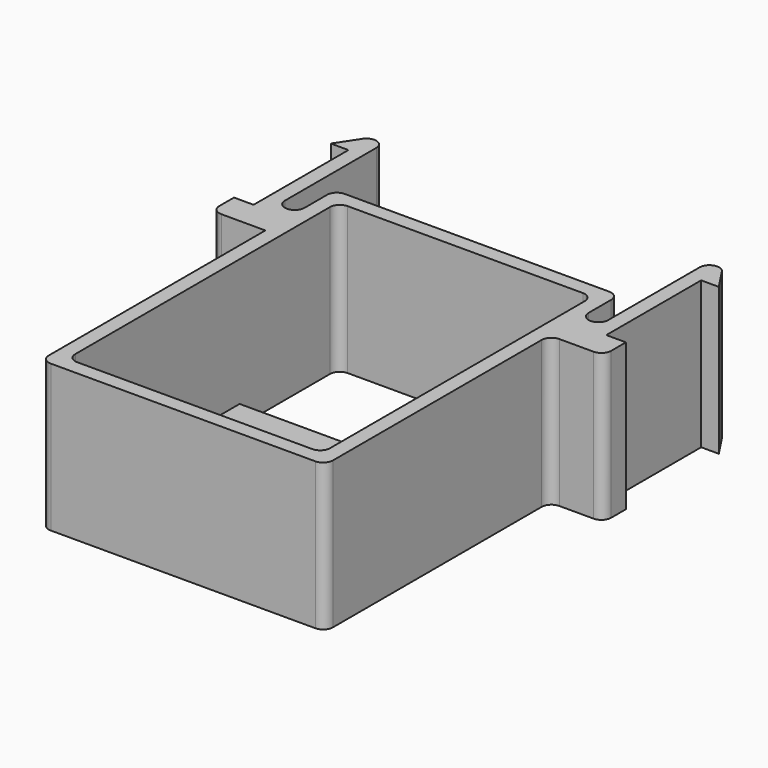
from build123d import *

# Parameters (mm, degrees)
F0_W     = 2
F0_H     = 4
F0_H_2   = 2.8740456328
F1_DEPTH = 15
F2_R     = 0.99999
F0_W_2   = 26
F0_H_3   = 7
F3_DEPTH = 2


# Not quite as in the source:
# - a fillet or chamfer is up to 0.001 mm smaller than in the source, because OpenCascade refuses the exact size


with BuildPart() as f1:
    # F0 (on Top) → F1 (new body)
    with BuildSketch(Plane.XY):
        Polygon((14.5, 18.75), (-14.5, 18.75), (-14.5, 13.8759543672), (-14.5, 9.8759543672), (-14.5, -18.75), (14.5, -18.75), (14.5, 9.8759543672), (14.5, 13.8759543672), align=None)
        Polygon((-13, 4.7144976147), (-13, 17.25), (13, 17.25), (13, 4.7144976147), (13, -2.2855023853), (13, -17.25), (-13, -17.25), (-13, -2.2855023853), align=None, mode=Mode.SUBTRACT)
        with Locations((-15.5, 11.8759543672)):
            Rectangle(F0_W, F0_H)
        Polygon((-16.5, 9.8759543672), (-16.5, 13.8759543672), (-16.5, 29.8609879265), (-19.8, 24.85), (-18, 24.85), (-18, 12.75), (-18, 9.8759543672), align=None)
        with Locations((15.5, 11.8759543672)):
            Rectangle(F0_W, F0_H)
        Polygon((16.5, 29.8609879265), (16.5, 13.8759543672), (16.5, 9.8759543672), (18, 9.8759543672), (18, 12.75), (18, 24.85), (19.8, 24.85), align=None)
        with Locations((-19, 11.3129771836)):
            Rectangle(F0_W, F0_H_2)
        with Locations((19, 11.3129771836)):
            Rectangle(F0_W, F0_H_2)
    extrude(amount=F1_DEPTH)

    # F2 (radius 1 in the source; OpenCascade refuses exactly that, so slightly less here)
    f2_edges = [f1.edges().sort_by_distance(p)[0] for p in [
        (-14.5, 18.75, 7.5),
        (-20, 9.875954, 7.5),
        (14.5, 18.75, 7.5),
        (20, 9.875954, 7.5),
        (-13, 17.25, 7.5),
        (14.5, 9.875954, 7.5),
        (14.5, -18.75, 7.5),
        (-14.5, -18.75, 7.5),
        (-13, -17.25, 7.5),
        (13, 17.25, 7.5),
        (13, -17.25, 7.5),
        (-14.5, 13.875954, 7.5),
        (16.5, 13.875954, 7.5),
        (-16.5, 13.875954, 7.5),
        (14.5, 13.875954, 7.5),
        (-16.5, 29.860988, 7.5),
        (16.5, 29.860988, 7.5),
    ]]
    fillet(f2_edges, radius=F2_R)

    # F0 (on Top) → F3 (join)
    with BuildSketch(Plane.XY):
        with Locations((0, 1.2144976147)):
            Rectangle(F0_W_2, F0_H_3)
    extrude(amount=F3_DEPTH)


solid = f1.part
